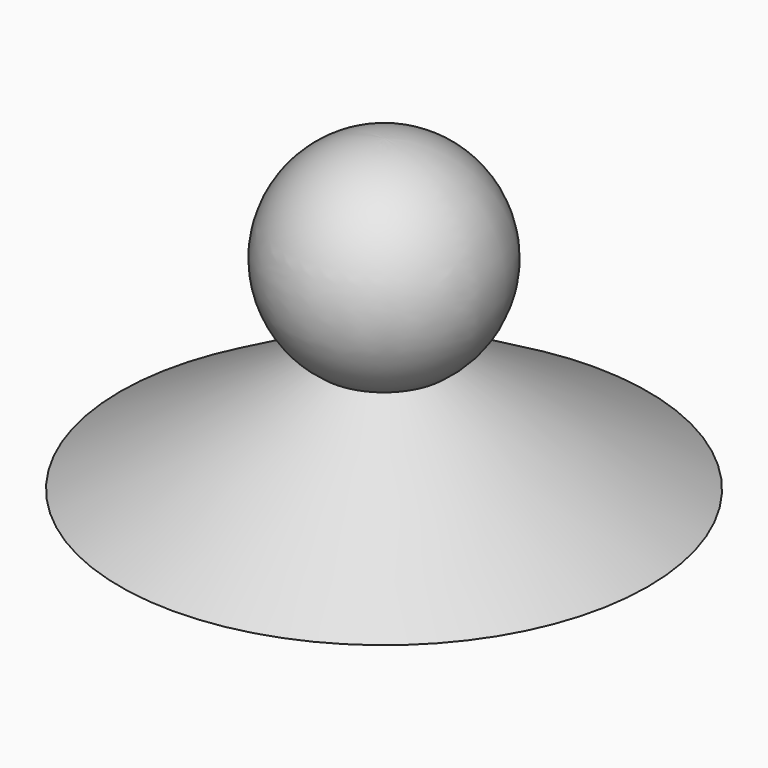
from build123d import *


# Not quite as in the source:
# - a feature names something its author has since deleted; it is built from what else it names


with BuildPart() as f1:
    # F0 (on Front) → F1 (revolve)
    with BuildSketch(Plane.XZ):
        Polygon((0, 11.43), (0, 0), (25.4, 0), (5.55625, 11.43), align=None)
    revolve(axis=Axis((0, 0, 5.715), (0, 0, 1)))

    # F2 (on Front) → F3 (revolve)
    with BuildSketch(Plane.XZ):
        with BuildLine():
            Line((0, 9.3980228781), (0, 29.7179276559))
            ThreePointArc((0, 29.7179276559), (-10.19110395, 19.557975267), (0, 9.3980228781))
        make_face()
    revolve(axis=Axis((0, 0, 17.444530502), (0, 0, 1)))


solid = f1.part
